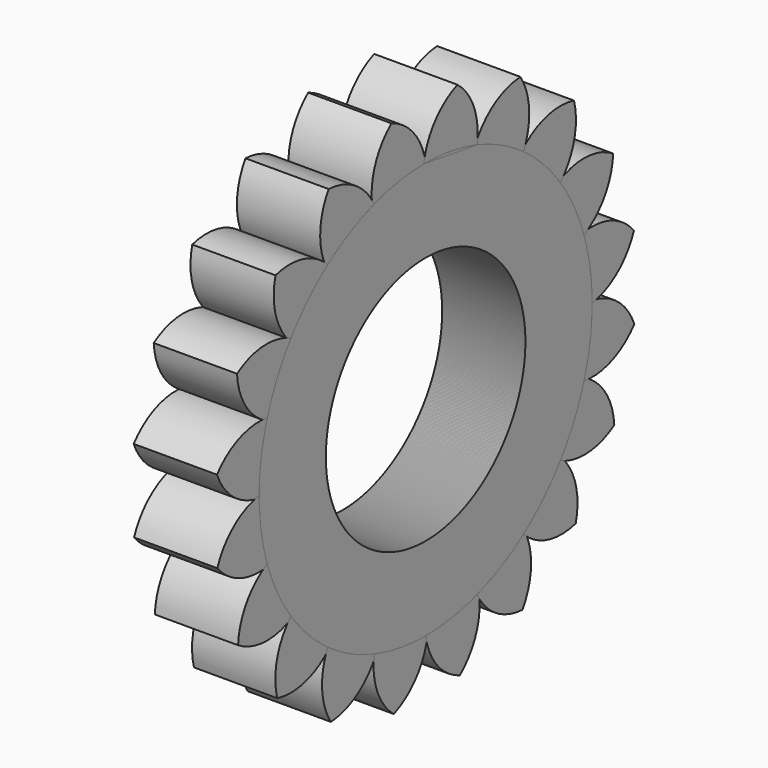
from build123d import *

# Parameters (mm, degrees)
F1_DEPTH = 12.7
F0_R     = 19.05
F2_COUNT = 20


with BuildPart() as f1:
    # F0 (on Right) → F1 (new body)
    with BuildSketch(Plane.YZ):
        with BuildLine():
            ThreePointArc((-10.16, 30.0805069771), (-5.1481260414, 31.3298467641), (0, 31.75))
            ThreePointArc((0, 31.75), (-2.195928409, 36.6063303464), (-6.5258233693, 39.714071591))
            ThreePointArc((-6.5258233693, 39.714071591), (-9.6335646139, 35.3841766307), (-10.16, 30.0805069771))
        make_face()
    extrude(amount=F1_DEPTH)


with BuildPart() as f1b:
    # F0 (on Right) → F1, piece 2 (new body)
    with BuildSketch(Plane.YZ):
        with BuildLine():
            ThreePointArc((-10.16, 30.0805069771), (-18.5132722661, -25.7938219347), (31.75, 0))
            ThreePointArc((31.75, 0), (22.4506403027, 22.4506403027), (0, 31.75))
            Line((0, 31.75), (-10.16, 30.0805069771))
        make_face()
        Circle(F0_R, mode=Mode.SUBTRACT)
    extrude(amount=F1_DEPTH)


with BuildPart() as f2_1:
    # F2: instance of F1
    add(f1.part.rotate(Axis((12.7, 0, 0), (1, 0, 0)), 1 * 360 / F2_COUNT))


with BuildPart() as f2_2:
    # F2: instance of F1
    add(f1.part.rotate(Axis((12.7, 0, 0), (1, 0, 0)), 2 * 360 / F2_COUNT))


with BuildPart() as f2_3:
    # F2: instance of F1
    add(f1.part.rotate(Axis((12.7, 0, 0), (1, 0, 0)), 3 * 360 / F2_COUNT))


with BuildPart() as f2_4:
    # F2: instance of F1
    add(f1.part.rotate(Axis((12.7, 0, 0), (1, 0, 0)), 4 * 360 / F2_COUNT))


with BuildPart() as f2_5:
    # F2: instance of F1
    add(f1.part.rotate(Axis((12.7, 0, 0), (1, 0, 0)), 5 * 360 / F2_COUNT))


with BuildPart() as f2_6:
    # F2: instance of F1
    add(f1.part.rotate(Axis((12.7, 0, 0), (1, 0, 0)), 6 * 360 / F2_COUNT))


with BuildPart() as f2_7:
    # F2: instance of F1
    add(f1.part.rotate(Axis((12.7, 0, 0), (1, 0, 0)), 7 * 360 / F2_COUNT))


with BuildPart() as f2_8:
    # F2: instance of F1
    add(f1.part.rotate(Axis((12.7, 0, 0), (1, 0, 0)), 8 * 360 / F2_COUNT))


with BuildPart() as f2_9:
    # F2: instance of F1
    add(f1.part.rotate(Axis((12.7, 0, 0), (1, 0, 0)), 9 * 360 / F2_COUNT))


with BuildPart() as f2_10:
    # F2: instance of F1
    add(f1.part.rotate(Axis((12.7, 0, 0), (1, 0, 0)), 10 * 360 / F2_COUNT))


with BuildPart() as f2_11:
    # F2: instance of F1
    add(f1.part.rotate(Axis((12.7, 0, 0), (1, 0, 0)), 11 * 360 / F2_COUNT))


with BuildPart() as f2_12:
    # F2: instance of F1
    add(f1.part.rotate(Axis((12.7, 0, 0), (1, 0, 0)), 12 * 360 / F2_COUNT))


with BuildPart() as f2_13:
    # F2: instance of F1
    add(f1.part.rotate(Axis((12.7, 0, 0), (1, 0, 0)), 13 * 360 / F2_COUNT))


with BuildPart() as f2_14:
    # F2: instance of F1
    add(f1.part.rotate(Axis((12.7, 0, 0), (1, 0, 0)), 14 * 360 / F2_COUNT))


with BuildPart() as f2_15:
    # F2: instance of F1
    add(f1.part.rotate(Axis((12.7, 0, 0), (1, 0, 0)), 15 * 360 / F2_COUNT))


with BuildPart() as f2_16:
    # F2: instance of F1
    add(f1.part.rotate(Axis((12.7, 0, 0), (1, 0, 0)), 16 * 360 / F2_COUNT))


with BuildPart() as f2_17:
    # F2: instance of F1
    add(f1.part.rotate(Axis((12.7, 0, 0), (1, 0, 0)), 17 * 360 / F2_COUNT))


with BuildPart() as f2_18:
    # F2: instance of F1
    add(f1.part.rotate(Axis((12.7, 0, 0), (1, 0, 0)), 18 * 360 / F2_COUNT))


with BuildPart() as f2_19:
    # F2: instance of F1
    add(f1.part.rotate(Axis((12.7, 0, 0), (1, 0, 0)), 19 * 360 / F2_COUNT))


with BuildPart() as f2_20:
    # F2: instance of F1b
    add(f1b.part.rotate(Axis((12.7, 0, 0), (1, 0, 0)), 1 * 360 / F2_COUNT))


with BuildPart() as f2_21:
    # F2: instance of F1b
    add(f1b.part.rotate(Axis((12.7, 0, 0), (1, 0, 0)), 2 * 360 / F2_COUNT))


with BuildPart() as f2_22:
    # F2: instance of F1b
    add(f1b.part.rotate(Axis((12.7, 0, 0), (1, 0, 0)), 3 * 360 / F2_COUNT))


with BuildPart() as f2_23:
    # F2: instance of F1b
    add(f1b.part.rotate(Axis((12.7, 0, 0), (1, 0, 0)), 4 * 360 / F2_COUNT))


with BuildPart() as f2_24:
    # F2: instance of F1b
    add(f1b.part.rotate(Axis((12.7, 0, 0), (1, 0, 0)), 5 * 360 / F2_COUNT))


with BuildPart() as f2_25:
    # F2: instance of F1b
    add(f1b.part.rotate(Axis((12.7, 0, 0), (1, 0, 0)), 6 * 360 / F2_COUNT))


with BuildPart() as f2_26:
    # F2: instance of F1b
    add(f1b.part.rotate(Axis((12.7, 0, 0), (1, 0, 0)), 7 * 360 / F2_COUNT))


with BuildPart() as f2_27:
    # F2: instance of F1b
    add(f1b.part.rotate(Axis((12.7, 0, 0), (1, 0, 0)), 8 * 360 / F2_COUNT))


with BuildPart() as f2_28:
    # F2: instance of F1b
    add(f1b.part.rotate(Axis((12.7, 0, 0), (1, 0, 0)), 9 * 360 / F2_COUNT))


with BuildPart() as f2_29:
    # F2: instance of F1b
    add(f1b.part.rotate(Axis((12.7, 0, 0), (1, 0, 0)), 10 * 360 / F2_COUNT))


with BuildPart() as f2_30:
    # F2: instance of F1b
    add(f1b.part.rotate(Axis((12.7, 0, 0), (1, 0, 0)), 11 * 360 / F2_COUNT))


with BuildPart() as f2_31:
    # F2: instance of F1b
    add(f1b.part.rotate(Axis((12.7, 0, 0), (1, 0, 0)), 12 * 360 / F2_COUNT))


with BuildPart() as f2_32:
    # F2: instance of F1b
    add(f1b.part.rotate(Axis((12.7, 0, 0), (1, 0, 0)), 13 * 360 / F2_COUNT))


with BuildPart() as f2_33:
    # F2: instance of F1b
    add(f1b.part.rotate(Axis((12.7, 0, 0), (1, 0, 0)), 14 * 360 / F2_COUNT))


with BuildPart() as f2_34:
    # F2: instance of F1b
    add(f1b.part.rotate(Axis((12.7, 0, 0), (1, 0, 0)), 15 * 360 / F2_COUNT))


with BuildPart() as f2_35:
    # F2: instance of F1b
    add(f1b.part.rotate(Axis((12.7, 0, 0), (1, 0, 0)), 16 * 360 / F2_COUNT))


with BuildPart() as f2_36:
    # F2: instance of F1b
    add(f1b.part.rotate(Axis((12.7, 0, 0), (1, 0, 0)), 17 * 360 / F2_COUNT))


with BuildPart() as f2_37:
    # F2: instance of F1b
    add(f1b.part.rotate(Axis((12.7, 0, 0), (1, 0, 0)), 18 * 360 / F2_COUNT))


with BuildPart() as f2_38:
    # F2: instance of F1b
    add(f1b.part.rotate(Axis((12.7, 0, 0), (1, 0, 0)), 19 * 360 / F2_COUNT))


solid = Compound([f1.part, f1b.part, f2_1.part, f2_2.part, f2_3.part, f2_4.part, f2_5.part, f2_6.part, f2_7.part, f2_8.part, f2_9.part, f2_10.part, f2_11.part, f2_12.part, f2_13.part, f2_14.part, f2_15.part, f2_16.part, f2_17.part, f2_18.part, f2_19.part, f2_20.part, f2_21.part, f2_22.part, f2_23.part, f2_24.part, f2_25.part, f2_26.part, f2_27.part, f2_28.part, f2_29.part, f2_30.part, f2_31.part, f2_32.part, f2_33.part, f2_34.part, f2_35.part, f2_36.part, f2_37.part, f2_38.part])
